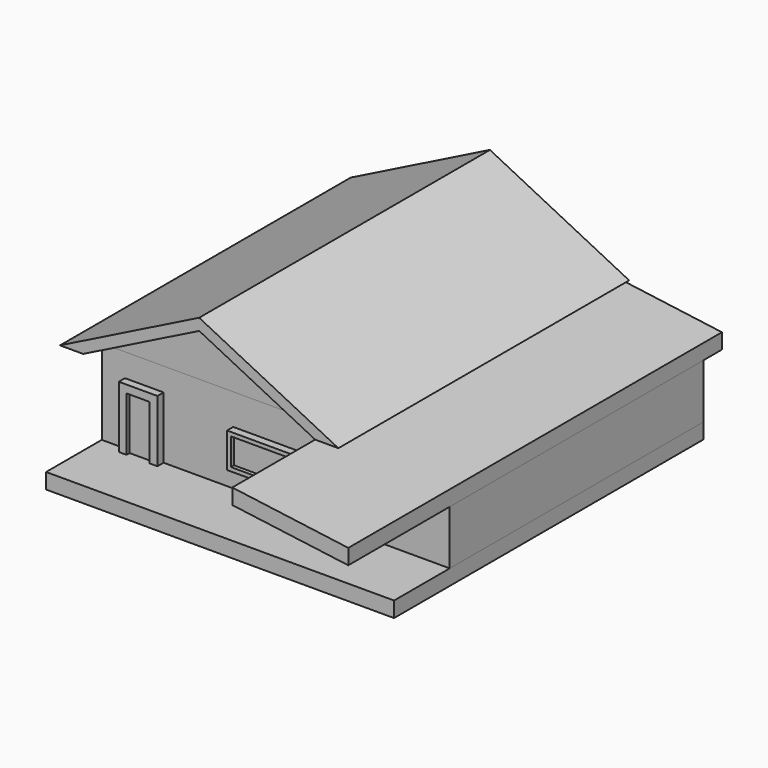
from build123d import *

# Parameters (mm, degrees)
F1_DEPTH      = 1219.2
F1_DEPTH_BACK = 13106.4
F2_DEPTH      = 304.8
F2_DEPTH_BACK = 12192
F0_W          = 4572
F0_H          = 609.6
F3_DEPTH      = 3048
F3_DEPTH_BACK = 12192
F0_W_2        = 2743.2
F0_H_2        = 1371.6
F0_W_3        = 1219.2
F0_W_4        = 2438.4
F0_H_3        = 1066.8
F0_W_5        = 914.4
F0_H_4        = 2133.6
F4_DEPTH      = 304.8
F4_DEPTH_BACK = 12192
F5_DEPTH      = 457.2
F6_DEPTH      = 609.6
F7_DEPTH      = 4084.32
F7_DEPTH_BACK = 30.48


with BuildPart() as f1:
    # F0 (on Front) → F1 (new body, two sides)
    with BuildSketch(Plane.XZ) as f1_sk:
        Polygon((-5486.4, 0), (-4572, 0), (0, 2286), (0, 2743.2), align=None)
        Polygon((0, 2286), (4572, 0), (5486.4, 0), (0, 2743.2), align=None)
    extrude(amount=F1_DEPTH)
    extrude(f1_sk.sketch, amount=-F1_DEPTH_BACK)



with BuildPart() as f1b:
    # F0 (on Front) → F1, piece 2 (new body, two sides)
    with BuildSketch(Plane.XZ) as f1_2_sk:
        Polygon((9144, -609.6), (4572, 0), (4572, -609.6), (9144, -1213.5698795319), align=None)
    extrude(amount=F1_DEPTH)
    extrude(f1_2_sk.sketch, amount=-F1_DEPTH_BACK)


with BuildPart() as f1_1:
    add(f1.part)

    add(f1b.part)  # F2 merges F1b
    # F0 (on Front) → F2 (join, two sides)
    with BuildSketch(Plane.XZ) as f2_sk:
        Polygon((-4572, 0), (0, 0), (0, 2286), align=None)
        Polygon((0, 2286), (0, 0), (4572, 0), align=None)
    extrude(amount=F2_DEPTH)
    extrude(f2_sk.sketch, amount=-F2_DEPTH_BACK)

    # F7 (add, two sides): a face of the model
    f7_faces = [f1_1.faces().sort_by_distance(p)[0] for p in [
        (6854.4648498046, -1219.2, -607.7232931773),
    ]]
    extrude(f7_faces, amount=F7_DEPTH)
    extrude(f7_faces, amount=-F7_DEPTH_BACK)


with BuildPart() as f3:
    # F0 (on Front) → F3 (new body, two sides)
    with BuildSketch(Plane.XZ) as f3_sk:
        Polygon((-3657.6, -3352.8), (-4572, -3352.8), (-4572, -3962.4), (4572, -3962.4), (4572, -3352.8), (-2133.6, -3352.8), (-2438.4, -3352.8), (-3352.8, -3352.8), align=None)
        with Locations((6858, -3657.6)):
            Rectangle(F0_W, F0_H)
    extrude(amount=F3_DEPTH)
    extrude(f3_sk.sketch, amount=-F3_DEPTH_BACK)


with BuildPart() as f4:
    # F0 (on Front) → F4 (new body, two sides)
    with BuildSketch(Plane.XZ) as f4_sk:
        Polygon((4572, 0), (0, 0), (-4572, 0), (-4572, -3352.8), (-3657.6, -3352.8), (-3657.6, -914.4), (-2133.6, -914.4), (-2133.6, -3352.8), (4572, -3352.8), (4572, -609.6), align=None)
        with Locations((1981.2, -1905)):
            Rectangle(F0_W_2, F0_H_2, mode=Mode.SUBTRACT)
        Polygon((9144, -1213.5698795319), (4572, -609.6), (4572, -3352.8), (9144, -3352.8), align=None)
        with Locations((6705.6, -1905)):
            Rectangle(F0_W_3, F0_H_2, mode=Mode.SUBTRACT)
        with Locations((1981.2, -1905)):
            Rectangle(F0_W_2, F0_H_2)
        with Locations((1981.2, -1905)):
            Rectangle(F0_W_4, F0_H_3, mode=Mode.SUBTRACT)
        with Locations((1981.2, -1905)):
            Rectangle(F0_W_4, F0_H_3)
        with Locations((-2895.6, -2286)):
            Rectangle(F0_W_5, F0_H_4)
        Polygon((-3657.6, -914.4), (-3657.6, -3352.8), (-3352.8, -3352.8), (-3352.8, -1219.2), (-2438.4, -1219.2), (-2438.4, -3352.8), (-2133.6, -3352.8), (-2133.6, -914.4), align=None)
        with Locations((6705.6, -1905)):
            Rectangle(F0_W_3, F0_H_2)
        with Locations((6705.6, -1905)):
            Rectangle(F0_W_5, F0_H_3, mode=Mode.SUBTRACT)
        with Locations((6705.6, -1905)):
            Rectangle(F0_W_5, F0_H_3)
    extrude(amount=F4_DEPTH)
    extrude(f4_sk.sketch, amount=-F4_DEPTH_BACK)


with BuildPart() as f5:
    # F0 (on Front) → F5 (new body)
    with BuildSketch(Plane.XZ):
        with Locations((-2895.6, -2286)):
            Rectangle(F0_W_5, F0_H_4)
    extrude(amount=F5_DEPTH)


with BuildPart() as f5b:
    # F0 (on Front) → F5, piece 2 (new body)
    with BuildSketch(Plane.XZ):
        with Locations((1981.2, -1905)):
            Rectangle(F0_W_4, F0_H_3)
    extrude(amount=F5_DEPTH)


with BuildPart() as f5c:
    # F0 (on Front) → F5, piece 3 (new body)
    with BuildSketch(Plane.XZ):
        with Locations((6705.6, -1905)):
            Rectangle(F0_W_5, F0_H_3)
    extrude(amount=F5_DEPTH)


with BuildPart() as f6:
    # F0 (on Front) → F6 (new body)
    with BuildSketch(Plane.XZ):
        Polygon((-3657.6, -914.4), (-3657.6, -3352.8), (-3352.8, -3352.8), (-3352.8, -1219.2), (-2438.4, -1219.2), (-2438.4, -3352.8), (-2133.6, -3352.8), (-2133.6, -914.4), align=None)
    extrude(amount=F6_DEPTH)


with BuildPart() as f6b:
    # F0 (on Front) → F6, piece 2 (new body)
    with BuildSketch(Plane.XZ):
        with Locations((1981.2, -1905)):
            Rectangle(F0_W_2, F0_H_2)
        with Locations((1981.2, -1905)):
            Rectangle(F0_W_4, F0_H_3, mode=Mode.SUBTRACT)
    extrude(amount=F6_DEPTH)


with BuildPart() as f6c:
    # F0 (on Front) → F6, piece 3 (new body)
    with BuildSketch(Plane.XZ):
        with Locations((6705.6, -1905)):
            Rectangle(F0_W_3, F0_H_2)
        with Locations((6705.6, -1905)):
            Rectangle(F0_W_5, F0_H_3, mode=Mode.SUBTRACT)
    extrude(amount=F6_DEPTH)


solid = Compound([f1_1.part, f3.part, f4.part, f5.part, f5b.part, f5c.part, f6.part, f6b.part, f6c.part])
